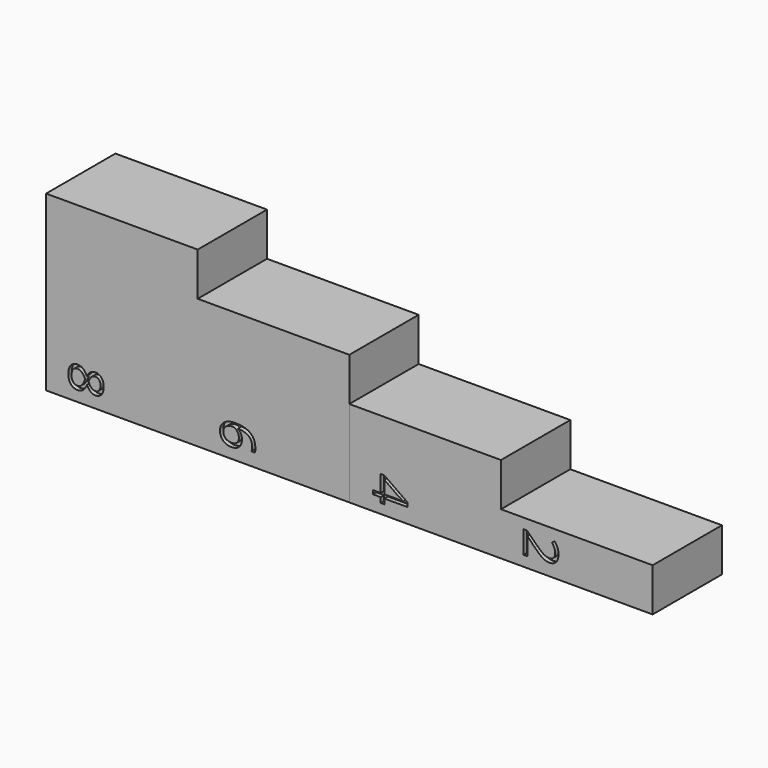
from build123d import *

# Parameters (mm, degrees)
F0_W         = 7
F0_H         = 4
F1_DEPTH     = 2
F2_DEPTH     = 4
F3_DEPTH     = 6
F4_DEPTH     = 8
F5_TEXT_SIZE = 2.2222222222
F6_DEPTH     = 0.2
F7_DEPTH     = 0.2


# Not quite as in the source:
# - Text() gives the source's letters only with a copy of the font that has no kerning and outlines rounded to 1/6400 em; it was checked with that copy


with BuildPart() as f1:
    # F0 (on Top) → F1 (new body)
    with BuildSketch(Plane.XY):
        with Locations((-15.5520305932, -3.8399192852)):
            Rectangle(F0_W, F0_H)
    extrude(amount=F1_DEPTH)

    # F0 (on Top) → F2 (join)
    with BuildSketch(Plane.XY):
        with Locations((-22.5520305932, -3.8399192852)):
            Rectangle(F0_W, F0_H)
    extrude(amount=F2_DEPTH)

    # F5 (on face) → F6 (cut)
    with BuildSketch(Plane.XZ.offset(5.8399192852)):
        with Locations(Location((-18.0042870343, 1.6377429105), (0, 0, -90))):
            Text('2', F5_TEXT_SIZE, font='Open Sans', text_align=(TextAlign.LEFT, TextAlign.BOTTOM))
        with Locations(Location((-24.9669607729, 1.6750692994), (0, 0, -90))):
            Text('4', F5_TEXT_SIZE, font='Open Sans', text_align=(TextAlign.LEFT, TextAlign.BOTTOM))
    extrude(amount=-F6_DEPTH, mode=Mode.SUBTRACT)


with BuildPart() as f3:
    # F0 (on Top) → F3 (new body)
    with BuildSketch(Plane.XY):
        with Locations((-29.5520305932, -3.8399192852)):
            Rectangle(F0_W, F0_H)
    extrude(amount=F3_DEPTH)

    # F0 (on Top) → F4 (join)
    with BuildSketch(Plane.XY):
        with Locations((-36.5520305932, -3.8399192852)):
            Rectangle(F0_W, F0_H)
    extrude(amount=F4_DEPTH)

    # F5 (on face) → F7 (cut)
    with BuildSketch(Plane.XZ.offset(5.8399192852)):
        with Locations(Location((-39.0022024512, 1.6398262438), (0, 0, -90))):
            Text('8', F5_TEXT_SIZE, font='Open Sans', text_align=(TextAlign.LEFT, TextAlign.BOTTOM))
        with Locations(Location((-31.9989062846, 1.6431248549), (0, 0, -90))):
            Text('6', F5_TEXT_SIZE, font='Open Sans', text_align=(TextAlign.LEFT, TextAlign.BOTTOM))
    extrude(amount=-F7_DEPTH, mode=Mode.SUBTRACT)


solid = Compound([f1.part, f3.part])
